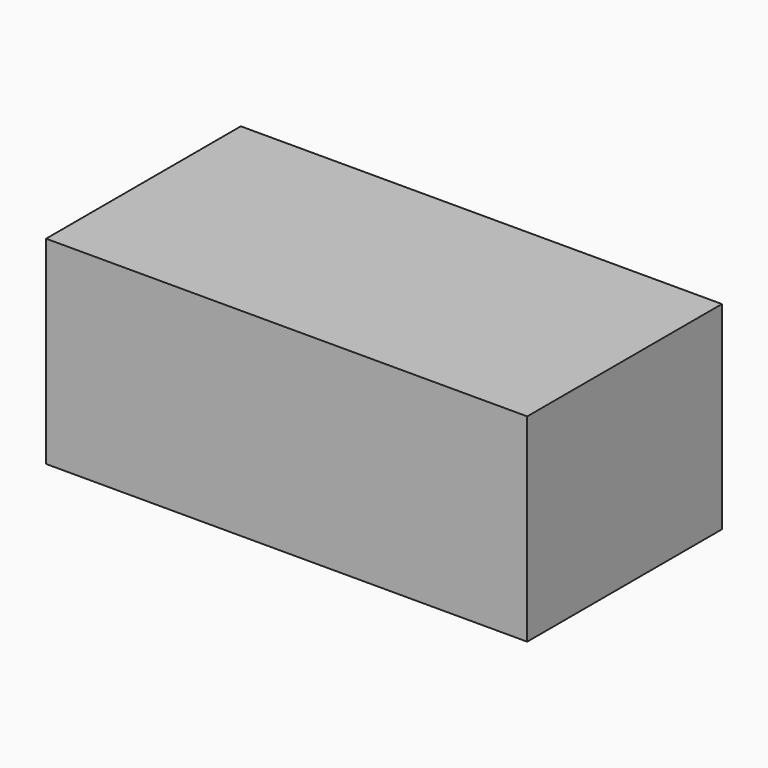
from build123d import *

# Parameters (mm, degrees)
F1_START = 22.352
F0_W     = 69.0019130707
F0_H     = 34.9036920816
F1_DEPTH = 28.448


# Not quite as in the source:
# - a feature names something its author has since deleted; it is built from what else it names


with BuildPart() as f1:
    # F0 (on Top) → F1 (new body)
    with BuildSketch(Plane.XY.offset(F1_START)):
        with Locations((-6.3095130026, 25.5065439269)):
            Rectangle(F0_W, F0_H)
    extrude(amount=F1_DEPTH)


solid = f1.part
